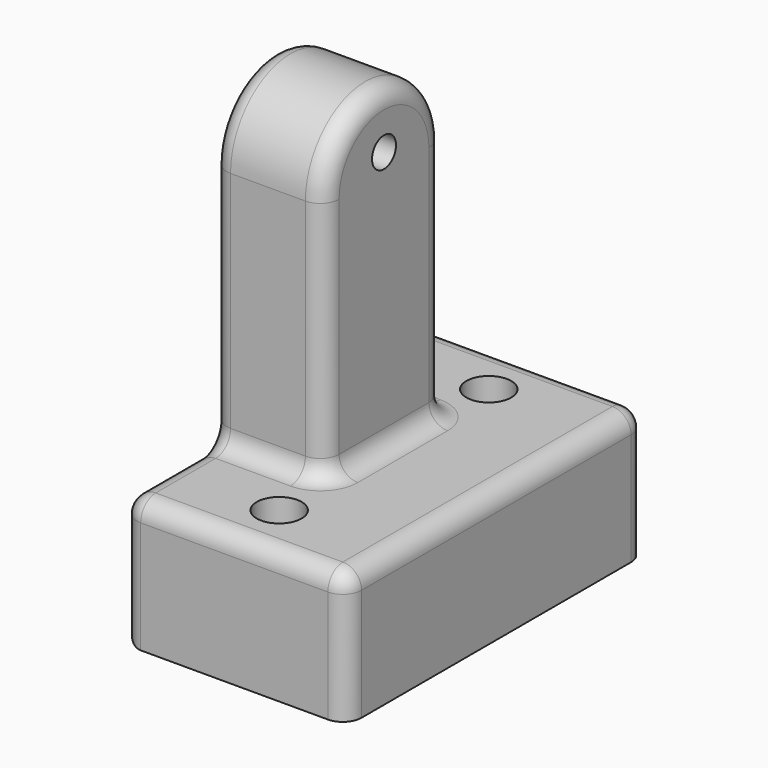
from build123d import *

# Parameters (mm, degrees)
F0_W     = 60
F0_H     = 100
F1_DEPTH = 100
F2_R     = 6
F3_DEPTH = 100
F4_R     = 6
F5_DEPTH = 65
F6_W     = 30
F6_H     = 20
F7_ANGLE = 180
F8_R     = 4
F9_DEPTH = 50
F10_R    = 5


with BuildPart() as f1:
    # F0 (on Top) → F1 (new body)
    with BuildSketch(Plane.XY):
        Rectangle(F0_W, F0_H)
    extrude(amount=F1_DEPTH)

    # F2 (on face) → F3 (cut)
    with BuildSketch(Plane.XY.offset(100)):
        with Locations((0, 35)):
            Circle(F2_R)
        with Locations((0, -35)):
            Circle(F2_R)
    extrude(amount=-F3_DEPTH, mode=Mode.SUBTRACT)

    # F4 (on face) → F5 (cut)
    with BuildSketch(Plane.XY.offset(100)):
        Polygon((0, 20), (0, 0), (0, -20), (-30, -20), (-30, -50), (30, -50), (30, 50), (-30, 50), (-30, 20), align=None)
        with Locations((0, -35)):
            Circle(F4_R, mode=Mode.SUBTRACT)
        with Locations((0, 35)):
            Circle(F4_R, mode=Mode.SUBTRACT)
    extrude(amount=-F5_DEPTH, mode=Mode.SUBTRACT)

    # F6 (on face) → F7 (revolve)
    with BuildSketch(Plane.XY.offset(100)):
        with Locations((-15, -10)):
            Rectangle(F6_W, F6_H)
    revolve(axis=Axis((-15, 0, 100), (-1, 0, 0)), revolution_arc=F7_ANGLE)

    # F8 (on face) → F9 (cut)
    with BuildSketch(Plane(origin=(-30, 0, 0), x_dir=(0, -1, 0), z_dir=(-1, 0, 0))):
        with Locations((0, 105)):
            Circle(F8_R)
    extrude(amount=-F9_DEPTH, mode=Mode.SUBTRACT)

    # F10
    f10_edges = [f1.edges().sort_by_distance(p)[0] for p in [
        (-30, 20, 67.5),
        (-30, 35, 35),
        (-30, 50, 17.5),
        (-30, 0, 0),
        (-30, -35, 35),
        (-30, -50, 17.5),
        (0, -50, 35),
        (30, -50, 17.5),
        (30, 0, 35),
        (-15, -20, 35),
        (0, -20, 67.5),
        (30, 50, 17.5),
        (0, 50, 35),
        (0, 0, 35),
        (-15, 20, 35),
        (-30, -20, 67.5),
        (-30, 0, 120),
        (0, 20, 67.5),
        (0, 0, 120),
    ]]
    fillet(f10_edges, radius=F10_R)


solid = f1.part
